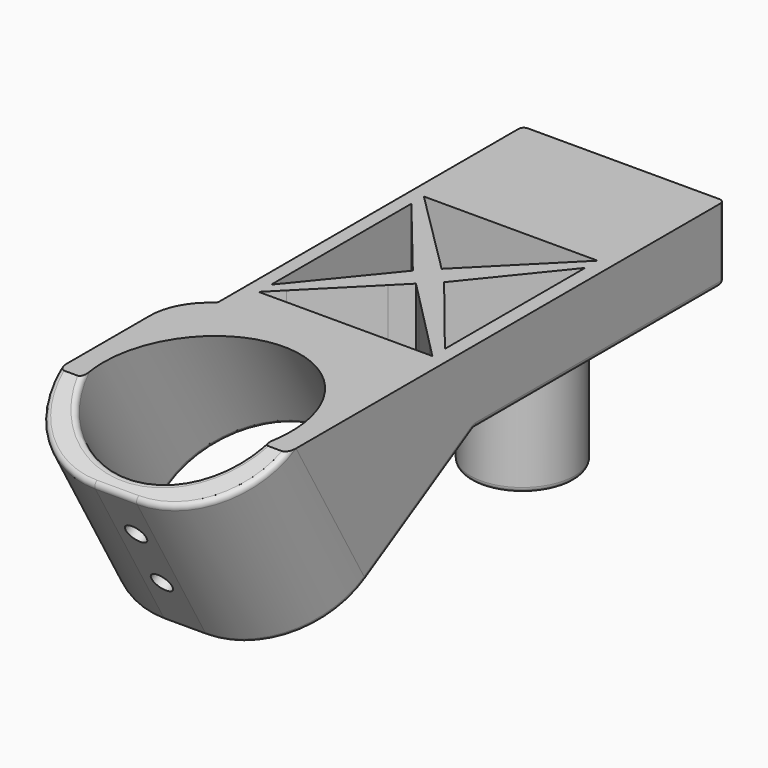
from build123d import *

# Parameters (mm, degrees)
F0_R      = 5
F1_DEPTH  = 16
F3_W      = 22
F3_H      = 30
F4_DEPTH  = 20
F6_W      = 22
F6_H      = 17.3205080757
F7_DEPTH  = 34
F10_D     = 18
F13_D     = 2
F13_DEPTH = 12
F13_TIP   = 0.600860619
F14_D     = 2
F14_DEPTH = 12
F14_TIP   = 0.600860619
F16_W     = 22
F16_H     = 40.5655099262
F17_DEPTH = 25
F18_R     = 9
F19_R     = 9
F21_DEPTH = 19
F22_R     = 0.5
F23_W     = 61.5093680099
F23_H     = 7.1933913681
F24_DEPTH = 25
F25_W     = 3
F25_H     = 1.5
F26_DEPTH = 25


with BuildPart() as f1:
    # F0 (on Top) → F1 (new body)
    with BuildSketch(Plane.XY):
        Circle(F0_R)
    extrude(amount=-F1_DEPTH)

    # F3 (on Top) → F4 (join)
    with BuildSketch(Plane.XY):
        with Locations((2, -7)):
            Rectangle(F3_W, F3_H)
    extrude(amount=F4_DEPTH)

    # F6 (on face) → F7 (join)
    with BuildSketch(Plane(origin=(0, -7.8397459622, -4.5262794416), x_dir=(-1, 0, 0), z_dir=(0, 0.8660254038, 0.5))):
        with Locations((-2, 19.6602540378)):
            Rectangle(F6_W, F6_H)
    extrude(amount=-F7_DEPTH)

    # F10 (through all)
    with Locations(Plane(origin=(0, -14.1602540378, 24.5262794416), x_dir=(1, 0, 0), z_dir=(0, -0.5, 0.8660254038))):
        with Locations((2, -32.3845669627)):
            Hole(F10_D / 2)

    # F13
    with Locations(Plane(origin=(0, -37.2846096908, -21.5262794416), x_dir=(1, 0, 0), z_dir=(0, -0.8660254038, -0.5))):
        with Locations((2, 16.8878287077)):
            Hole(F13_D / 2, depth=F13_DEPTH)
            with Locations((0, 0, -(F13_DEPTH + F13_TIP / 2))):  # 118° drill point
                Cone(0, F13_D / 2, F13_TIP, mode=Mode.SUBTRACT)

    # F14
    with Locations(Plane(origin=(0, -37.2846096908, -21.5262794416), x_dir=(1, 0, 0), z_dir=(0, -0.8660254038, -0.5))):
        with Locations((2, 23.0905413628)):
            Hole(F14_D / 2, depth=F14_DEPTH)
            with Locations((0, 0, -(F14_DEPTH + F14_TIP / 2))):  # 118° drill point
                Cone(0, F14_D / 2, F14_TIP, mode=Mode.SUBTRACT)

    # F16 (on offset) → F17 (cut)
    with BuildSketch(Plane.XY.offset(13.9)):
        with Locations((2, -12.2827549631)):
            Rectangle(F16_W, F16_H)
    extrude(amount=F17_DEPTH, mode=Mode.SUBTRACT)

    # F18
    f18_edges = [f1.edges().sort_by_distance(p)[0] for p in [
        (-9, -47.114737, -4.5),
    ]]
    fillet(f18_edges, radius=F18_R)

    # F19
    f19_edges = [f1.edges().sort_by_distance(p)[0] for p in [
        (13, -47.114737, -4.5),
    ]]
    fillet(f19_edges, radius=F19_R)

    # F20 (on face) → F21 (cut, symmetric)
    with BuildSketch(Plane(origin=(0, 0, 0), x_dir=(1, 0, 0), z_dir=(0, 0, -1))):
        with BuildLine():
            Line((-9, 33.4308072925), (-9, -8))
            Line((-9, -8), (-6.3705204485, -8))
            Line((-6.3705204485, -8), (-6.3705204485, 28.6556702479))
            ThreePointArc((-6.3705204485, 28.6556702479), (-8.2991685647, 30.7051836709), (-9, 33.4308072925))
        make_face()
    extrude(amount=F21_DEPTH, both=True, mode=Mode.SUBTRACT)

    # F22
    f22_edges = [f1.edges().sort_by_distance(p)[0] for p in [
        (-6.363961, -49.161987, 4.318019),
        (-8.07524, -30.333122, 13.9),
        (13, -12.282755, 13.9),
        (2.033323, -32.56551, 13.9),
        (-6.37052, -10.327835, 13.9),
        (3.31474, 8, 13.9),
        (-6.37052, 8, 6.95),
        (-6.37052, -7, 0),
        (-6.37052, -25.327835, -1.921327),
        (-6.37052, -28.65567, 5.028673),
        (13, -7, 0),
        (3.31474, -22, 0),
        (3.31474, 8, 0),
        (-5, 0, 0),
        (13, 8, 6.95),
        (5, 0, -8),
        (-5, 0, -16),
        (10.363961, -40.501733, -10.681981),
        (13, -28.495191, -3.75),
        (-8.299169, -30.705184, -5.02594),
        (-9, -34.210594, -7.04979),
        (-6.363961, -40.501733, -10.681981),
        (2, -42.78461, -12),
        (-7, -33.545858, -6.666004),
        (10.363961, -49.161987, 4.318019),
        (2, -51.444864, 3),
        (-7, -42.206112, 8.333996),
    ]]
    fillet(f22_edges, radius=F22_R)

    # F23 (on face) → F24 (cut)
    with BuildSketch(Plane.YZ.offset(13)):
        with Locations((-17.0258260332, 10.6636829822)):
            Rectangle(F23_W, F23_H)
    extrude(amount=-F24_DEPTH, mode=Mode.SUBTRACT)

    # F25 (on face) → F26 (cut)
    with BuildSketch(Plane.XY.offset(7.0669872981)):
        Polygon((-3.5632000846, -23.8186163443), (-5.0563900732, -25.3186163443), (1.8147397757, -25.3186163443), (1.8147397757, -23.8186163443), align=None)
        Polygon((-5.0563900732, -7), (-5.0563900732, -23.8186163443), (1.8147397757, -15.4093081722), align=None)
        Polygon((1.8147397757, -18.4161492421), (-3.5632000846, -23.8186163443), (1.8147397757, -23.8186163443), align=None)
        with Locations((3.3147397757, -24.5686163443)):
            Rectangle(F25_W, F25_H)
        Polygon((3.3147397757, -16.9093081722), (1.8147397757, -18.4161492421), (1.8147397757, -23.8186163443), (4.8147397757, -23.8186163443), (4.8147397757, -18.4288208692), align=None)
        Polygon((4.8147397757, -23.8186163443), (4.8147397757, -25.3186163443), (11.6160605103, -25.3186163443), (10.1353226366, -23.8186163443), align=None)
        Polygon((1.8147397757, -5.5), (-5.0563900732, -5.5), (-3.5495490032, -7), (1.8147397757, -7), align=None)
        Polygon((1.8147397757, -7), (-3.5495490032, -7), (1.8147397757, -12.3399348669), align=None)
        Polygon((1.8147397757, -7), (1.8147397757, -12.3399348669), (3.3147397757, -13.8331248555), (4.8147397757, -12.3273780373), (4.8147397757, -7), align=None)
        Polygon((4.8147397757, -18.4288208692), (4.8147397757, -23.8186163443), (10.1353226366, -23.8186163443), align=None)
        with Locations((3.3147397757, -6.25)):
            Rectangle(F25_W, F25_H)
        Polygon((4.8147397757, -15.4093081722), (11.6160605103, -23.8186163443), (11.6160605103, -7), align=None)
        Polygon((11.6160605103, -5.5), (4.8147397757, -5.5), (4.8147397757, -7), (10.1217853953, -7), align=None)
        Polygon((10.1217853953, -7), (4.8147397757, -7), (4.8147397757, -12.3273780373), align=None)
    extrude(amount=-F26_DEPTH, mode=Mode.SUBTRACT)


solid = f1.part
